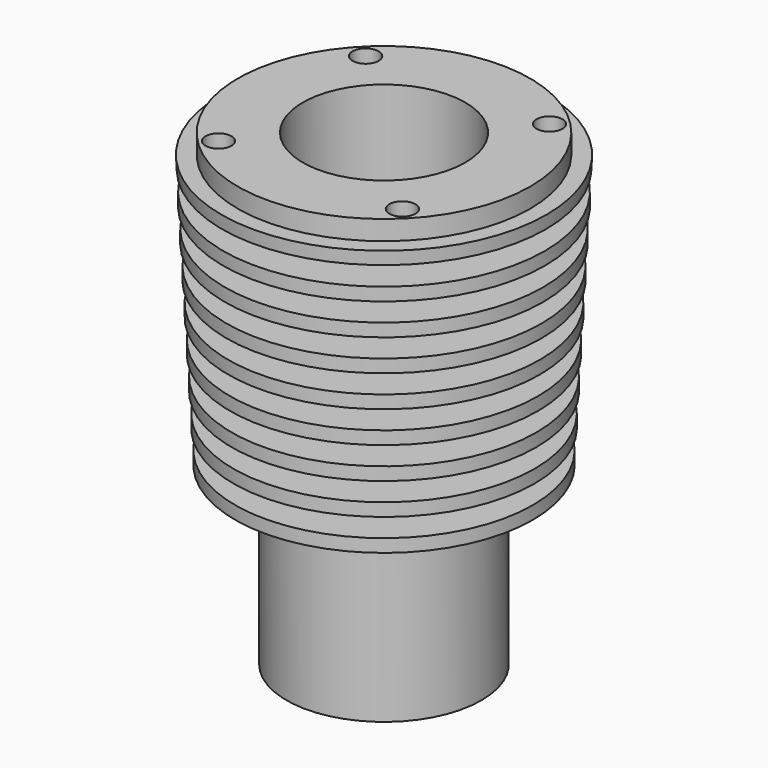
from build123d import *

# Parameters (mm, degrees)
F2_R            = 50.8
F3_DEPTH        = 127
F3_COPIES_COUNT = 4


# Not quite as in the source:
# - a pattern or mirror of a feature is missing from the dataset's text; its kind, count and spacing are read off the source's solid


with BuildPart() as f1:
    # F0 (on Front) → F1 (revolve)
    with BuildSketch(Plane.XZ):
        with BuildLine():
            Line((571.5, -76.2), (317.5, -76.2))
            Line((317.5, -76.2), (317.5, -1828.8))
            Line((317.5, -1828.8), (381, -1828.8))
            Line((381, -1828.8), (381, -1651))
            Line((381, -1651), (381, -1524))
            Line((381, -1524), (381, -1143))
            Line((381, -1143), (444.5, -1143))
            Line((444.5, -1143), (579.0913810609, -1143))
            Line((579.0913810609, -1143), (581.7536962484, -1143))
            Line((581.7536962484, -1143), (581.7536962484, -1092.2))
            Line((581.7536962484, -1092.2), (444.5, -1092.2))
            ThreePointArc((444.5, -1092.2), (406.4, -1054.1), (444.5, -1016))
            Line((444.5, -1016), (588.4094842174, -1016))
            Line((588.4094842174, -1016), (588.4094842174, -965.2))
            Line((588.4094842174, -965.2), (444.5, -965.2))
            ThreePointArc((444.5, -965.2), (406.4, -927.1), (444.5, -889))
            Line((444.5, -889), (595.0652721863, -889))
            Line((595.0652721863, -889), (595.0652721863, -838.2))
            Line((595.0652721863, -838.2), (444.5, -838.2))
            ThreePointArc((444.5, -838.2), (406.4, -800.1), (444.5, -762))
            Line((444.5, -762), (601.7210601553, -762))
            Line((601.7210601553, -762), (601.7210601553, -711.2))
            Line((601.7210601553, -711.2), (444.5, -711.2))
            ThreePointArc((444.5, -711.2), (406.4, -673.1), (444.5, -635))
            Line((444.5, -635), (608.3768481242, -635))
            Line((608.3768481242, -635), (608.3768481242, -584.2))
            Line((608.3768481242, -584.2), (444.5, -584.2))
            ThreePointArc((444.5, -584.2), (406.4, -546.1), (444.5, -508))
            Line((444.5, -508), (615.0326360932, -508))
            Line((615.0326360932, -508), (615.0326360932, -457.2))
            Line((615.0326360932, -457.2), (444.5, -457.2))
            ThreePointArc((444.5, -457.2), (406.4, -419.1), (444.5, -381))
            Line((444.5, -381), (621.6884240621, -381))
            Line((621.6884240621, -381), (621.6884240621, -330.2))
            Line((621.6884240621, -330.2), (444.5, -330.2))
            ThreePointArc((444.5, -330.2), (406.4, -292.1), (444.5, -254))
            Line((444.5, -254), (628.3442120311, -254))
            Line((628.3442120311, -254), (628.3442120311, -203.2))
            Line((628.3442120311, -203.2), (444.5, -203.2))
            ThreePointArc((444.5, -203.2), (406.4, -165.1), (444.5, -127))
            Line((444.5, -127), (632.3376848124, -127))
            Line((632.3376848124, -127), (635, -76.2))
            Line((635, -76.2), (571.5, -76.2))
        make_face()
        Polygon((381, 0), (317.5, 0), (317.5, -76.2), (571.5, -76.2), (571.5, 0), align=None)
    revolve(axis=Axis((0, 0, -597.5417420604), (0, 0, -1)))

    # F2 (on Top) → F3 (cut, through all)
    with BuildSketch(Plane.XY):
        with Locations((-359.2102448428, -359.2102448428)):
            Circle(F2_R)
    f3 = extrude(amount=-F3_DEPTH, mode=Mode.SUBTRACT)

    # F3_copies: F3 ×4 about axis
    f3_copies_axis = Axis((0, 0, 0), (0, 0, 1))
    for i in range(1, F3_COPIES_COUNT):
        add(f3.rotate(f3_copies_axis, i * 360 / F3_COPIES_COUNT), mode=Mode.SUBTRACT)


solid = f1.part
